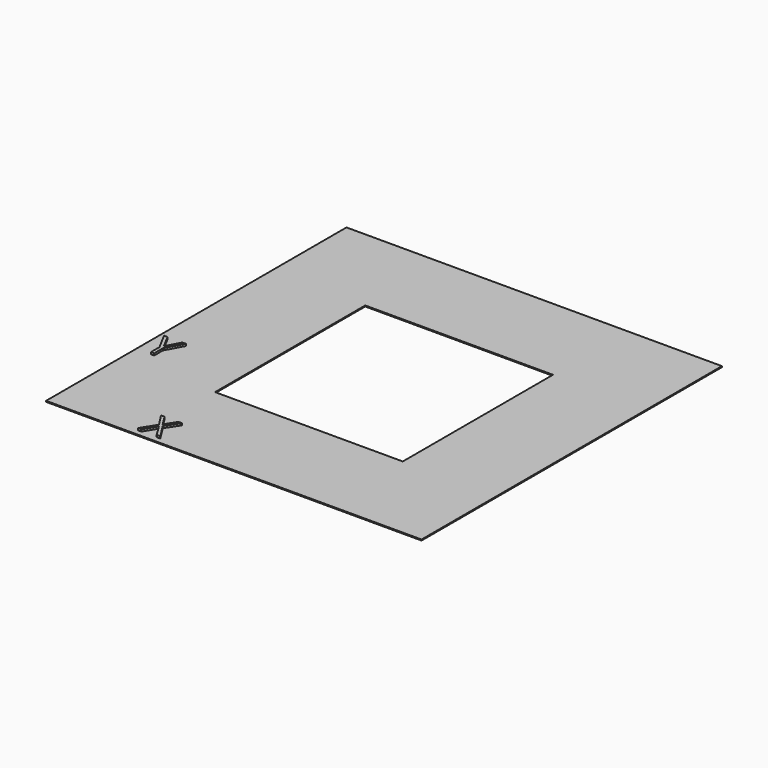
from build123d import *

# Parameters (mm, degrees)
F0_W         = 100
F0_H         = 100
F0_W_2       = 50
F0_H_2       = 50
F1_DEPTH     = 0.2625
F2_TEXT_SIZE = 10.4487666653
F3_DEPTH     = 0.525


# Not quite as in the source:
# - Text() gives the source's letters only with a copy of the font that has no kerning and outlines rounded to 1/6400 em; it was checked with that copy


with BuildPart() as f1:
    # F0 (on Top) → F1 (new body)
    with BuildSketch(Plane.XY):
        with Locations((14.28270787, -7.3281310499)):
            Rectangle(F0_W, F0_H)
        with Locations((14.28270787, -7.3281310499)):
            Rectangle(F0_W_2, F0_H_2, mode=Mode.SUBTRACT)
    extrude(amount=F1_DEPTH)

    # F2 (on face) → F3 (join)
    with BuildSketch(Plane.XY.offset(0.2625)):
        with Locations((-34.2535031959, -27.3493174464)):
            Text('Y', F2_TEXT_SIZE, font='Open Sans', text_align=(TextAlign.LEFT, TextAlign.BOTTOM))
        with Locations((-12.5331294904, -55.769962776)):
            Text('X', F2_TEXT_SIZE, font='Open Sans', text_align=(TextAlign.LEFT, TextAlign.BOTTOM))
    extrude(amount=F3_DEPTH)


solid = f1.part
